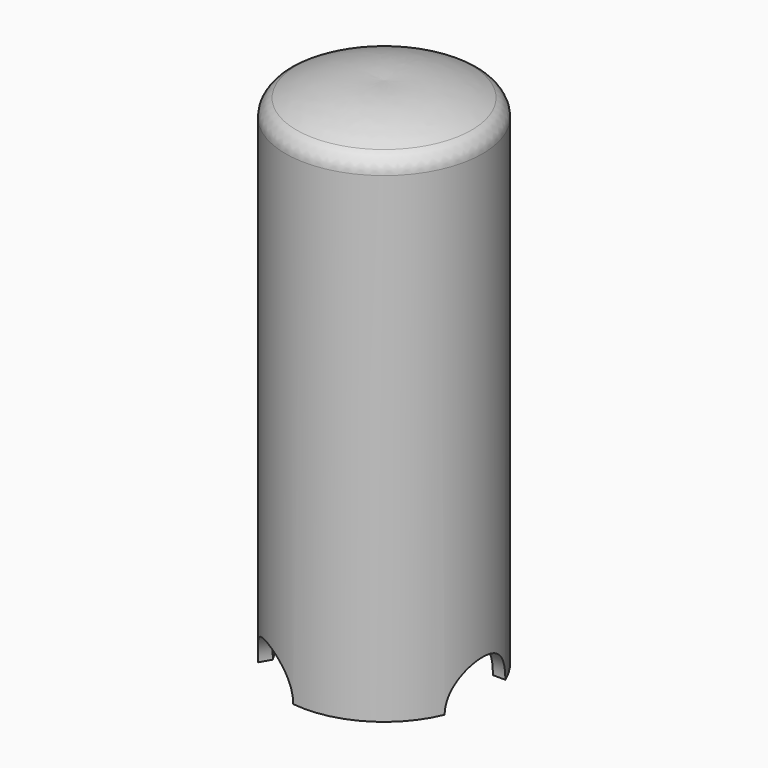
from build123d import *

# Parameters (mm, degrees)
F2_R            = 5
F4_R            = 10
F5_DEPTH        = 30
F5_COPIES_COUNT = 3


# Not quite as in the source:
# - a pattern or mirror of a feature is missing from the dataset's text; its kind, count and spacing are read off the source's solid


with BuildPart() as f1:
    # F0 (on Front) → F1 (revolve)
    with BuildSketch(Plane.XZ):
        with BuildLine():
            Line((-26, 0), (-23, 0))
            Line((-23, 0), (-23, 130))
            ThreePointArc((-23, 130), (-11.6527720396, 132.6534483777), (0, 132.5382334783))
            Line((0, 132.5382334783), (0, 135.5382334783))
            ThreePointArc((0, 135.5382334783), (-13.4057477437, 134.6739554169), (-26, 130))
            Line((-26, 130), (-26, 0))
        make_face()
    revolve(axis=Axis((0, 0, 8.4112687036), (0, 0, 1)))

    # F2
    f2_edges = [f1.edges().sort_by_distance(p)[0] for p in [
        (26, 0, 130),
    ]]
    fillet(f2_edges, radius=F2_R)

    # F4 (on offset) → F5 (cut)
    with BuildSketch(Plane.YZ.offset(40)):
        Circle(F4_R)
    f5 = extrude(amount=-F5_DEPTH, mode=Mode.SUBTRACT)

    # F5_copies: F5 ×3 about axis
    f5_copies_axis = Axis((0, 0, 0), (0, 0, 1))
    for i in range(1, F5_COPIES_COUNT):
        add(f5.rotate(f5_copies_axis, i * 360 / F5_COPIES_COUNT), mode=Mode.SUBTRACT)


solid = f1.part
